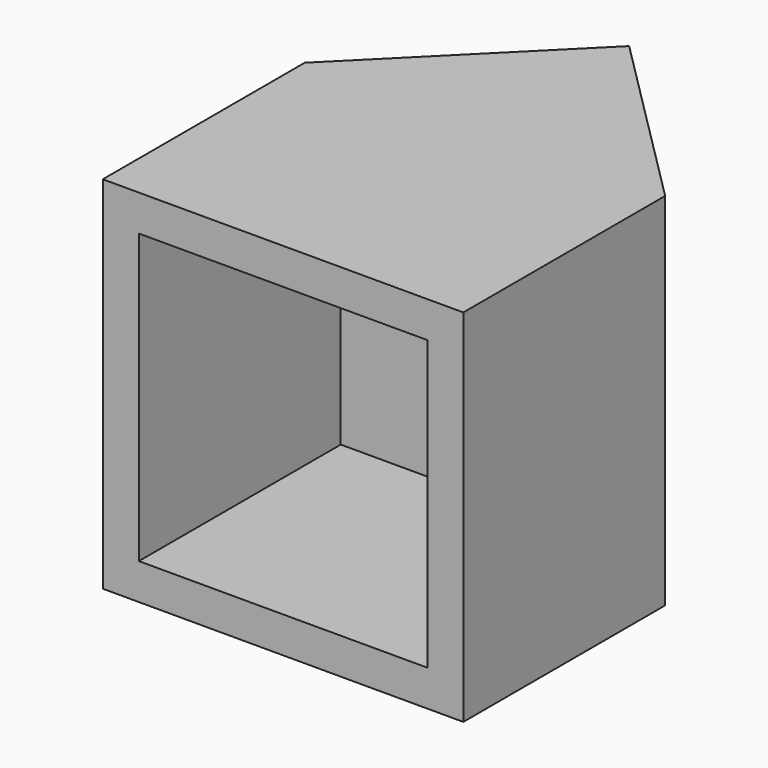
from build123d import *

# Parameters (mm, degrees)
F0_W     = 50
F0_H     = 50
F0_W_2   = 40
F0_H_2   = 40
F1_DEPTH = 35
F2_W     = 50
F2_H     = 50
F3_DEPTH = 25
F4_SIZE  = 24.99999


# Not quite as in the source:
# - a fillet or chamfer is up to 0.001 mm smaller than in the source, because OpenCascade refuses the exact size


with BuildPart() as f1:
    # F0 (on Front) → F1 (new body)
    with BuildSketch(Plane.XZ):
        with Locations((25, 25)):
            Rectangle(F0_W, F0_H)
        with Locations((25, 25)):
            Rectangle(F0_W_2, F0_H_2, mode=Mode.SUBTRACT)
    extrude(amount=-F1_DEPTH)

    # F2 (on face) → F3 (join)
    with BuildSketch(Plane(origin=(0, 35, 0), x_dir=(-1, 0, 0), z_dir=(0, 1, 0))):
        with Locations((-25, 25)):
            Rectangle(F2_W, F2_H)
    extrude(amount=F3_DEPTH)

    # F4 (size 25 in the source; OpenCascade refuses exactly that, so slightly less here)
    f4_edges = [f1.edges().sort_by_distance(p)[0] for p in [
        (0, 60, 25),
        (50, 60, 25),
    ]]
    chamfer(f4_edges, length=F4_SIZE)


solid = f1.part
